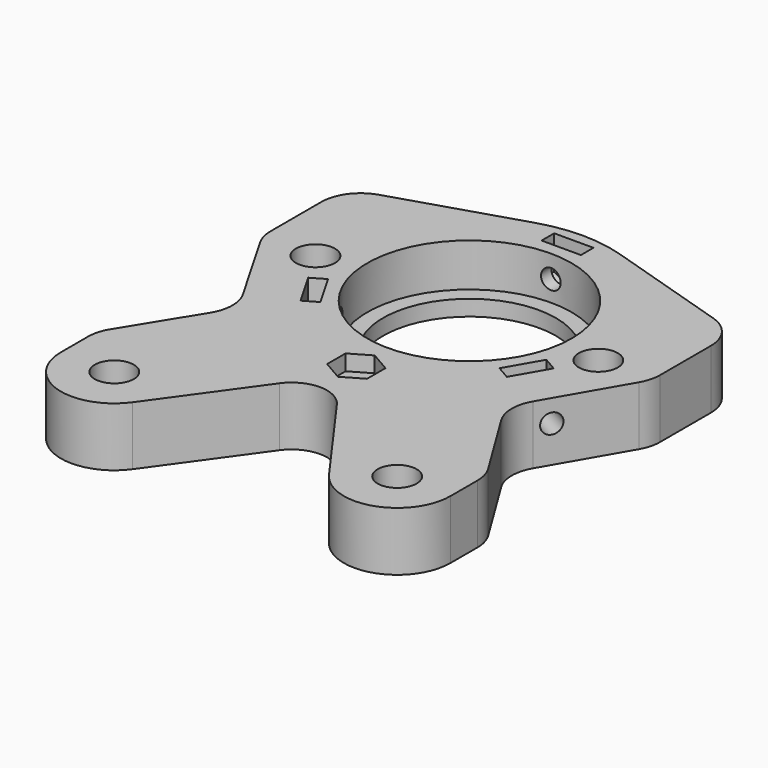
from build123d import *

# Parameters (mm, degrees)
F0_R        = 3.1496
F0_R_2      = 16.51
F1_DEPTH    = 9.525
F0_R_3      = 13.97
F2_DEPTH    = 2.54
F4_DEPTH    = 8.636
F5_T1_DEPTH = 2.54
F5_T3_DEPTH = 2.54
F5_T5_DEPTH = 2.54
F5_T7_DEPTH = 2.54
F5_T9_DEPTH = 2.54
F6_R        = 1.5875
F9_DEPTH    = 5.08
F7_R        = 1.5875
F10_DEPTH   = 20.32
F8_R        = 1.5875
F11_DEPTH   = 20.32
F13_DEPTH   = 2.54


# Not quite as in the source:
# - a fillet or chamfer that OpenCascade refuses, or shapes differently, is made with other operations: its cross-section is extruded or revolved along the edge and cut away or added
# - a feature names something its author has since deleted; it is built from what else it names


with BuildPart() as f1:
    # F0 (on Top) → F1 (new body)
    with BuildSketch(Plane.XY):
        with BuildLine():
            ThreePointArc((6.8331158271, 57.7357942584), (0, 58.780934), (-6.8331158271, 57.7357942584))
            Line((-6.8331158271, 57.7357942584), (-27.0242026981, 51.4112964789))
            ThreePointArc((-27.0242026981, 51.4112964789), (-30.2435047856, 49.1112435687), (-31.4761149683, 45.3516130738))
            Line((-31.4761149683, 45.3516130738), (-31.4761149683, 35.0824113719))
            ThreePointArc((-31.4761149683, 35.0824113719), (-31.2597439653, 33.4389104355), (-30.6253762824, 31.9074113719))
            Line((-30.6253762824, 31.9074113719), (-23.4250291837, 19.436044365))
            ThreePointArc((-23.4250291837, 19.436044365), (-22.5749179632, 16.1717783736), (-23.516459851, 12.9327012793))
            Line((-23.516459851, 12.9327012793), (-30.5339456151, 1.5308194413))
            ThreePointArc((-30.5339456151, 1.5308194413), (-31.2360341416, -0.0679607815), (-31.4761149683, -1.7975236443))
            Line((-31.4761149683, -1.7975236443), (-31.4761149683, -7.259066))
            ThreePointArc((-31.4761149683, -7.259066), (-25.5004563551, -15.4606163037), (-15.8622501042, -12.2858874155))
            Line((-15.8622501042, -12.2858874155), (-4.6415514186, 3.3342503548))
            ThreePointArc((-4.6415514186, 3.3342503548), (0, 5.715), (4.6415514186, 3.3342503548))
            Line((4.6415514186, 3.3342503548), (15.8622501042, -12.2858874155))
            ThreePointArc((15.8622501042, -12.2858874155), (25.5004563551, -15.4606163037), (31.4761149683, -7.259066))
            Line((31.4761149683, -7.259066), (31.4761149683, -1.7975236443))
            ThreePointArc((31.4761149683, -1.7975236443), (31.2360341416, -0.0679607815), (30.5339456151, 1.5308194413))
            Line((30.5339456151, 1.5308194413), (23.516459851, 12.9327012793))
            ThreePointArc((23.516459851, 12.9327012793), (22.5749179632, 16.1717783736), (23.4250291837, 19.436044365))
            Line((23.4250291837, 19.436044365), (30.6253762824, 31.9074113719))
            ThreePointArc((30.6253762824, 31.9074113719), (31.2597439653, 33.4389104355), (31.4761149683, 35.0824113719))
            Line((31.4761149683, 35.0824113719), (31.4761149683, 45.3516130738))
            ThreePointArc((31.4761149683, 45.3516130738), (30.2435047856, 49.1112435687), (27.0242026981, 51.4112964789))
            Line((27.0242026981, 51.4112964789), (6.8331158271, 57.7357942584))
        make_face()
        with Locations((-22.86, -7.259066)):
            Circle(F0_R, mode=Mode.SUBTRACT)
        with Locations((22.86, -7.259066)):
            Circle(F0_R, mode=Mode.SUBTRACT)
        with Locations((-22.86, 33.380934)):
            Circle(F0_R, mode=Mode.SUBTRACT)
        with Locations((0, 35.920934)):
            Circle(F0_R_2, mode=Mode.SUBTRACT)
        with Locations((22.86, 33.380934)):
            Circle(F0_R, mode=Mode.SUBTRACT)
    extrude(amount=F1_DEPTH)

    # F0 (on Top) → F2 (join)
    with BuildSketch(Plane.XY):
        with Locations((0, 35.920934)):
            Circle(F0_R_2)
        with Locations((0, 35.920934)):
            Circle(F0_R_3, mode=Mode.SUBTRACT)
    extrude(amount=F2_DEPTH)

    # F3 (on face) → F4 (cut)
    with BuildSketch(Plane.XY.offset(9.525)):
        Polygon((17.6453415423, 29.39956552), (14.4703415423, 23.900304206), (16.6700460679, 22.630304206), (19.8450460679, 28.12956552), align=None)
        Polygon((-3.175, 57.002932274), (-3.175, 54.462932274), (0, 54.462932274), (3.175, 54.462932274), (3.175, 57.002932274), align=None)
        Polygon((-14.4703415423, 23.900304206), (-17.6453415423, 29.39956552), (-19.8450460679, 28.12956552), (-16.6700460679, 22.630304206), align=None)
    extrude(amount=-F4_DEPTH, mode=Mode.SUBTRACT)

    # F5: chamfer of 3.175 x 5.499261314 on 6 edges, made by hand

    # F5_s2 → F5_t1 (join)
    with BuildSketch(Plane(origin=(-0.5036208564, -0.290765637, 0), x_dir=(0, 0, 1), z_dir=(-0.8660254038, -0.5, 0))):
        Polygon((4.064, 34.2834413717), (0.889, 28.7841800576), (0.889, 34.2834413717), align=None)
    extrude(amount=F5_T1_DEPTH)

    # F5_s4 → F5_t3 (join)
    with BuildSketch(Plane(origin=(-2.703325382, -1.560765637, 0), x_dir=(0, 0, 1), z_dir=(0.8660254038, 0.5, 0))):
        Polygon((4.064, -27.9334413717), (0.889, -33.4327026857), (0.889, -27.9334413717), align=None)
    extrude(amount=F5_T3_DEPTH)

    # F5_s6 → F5_t5 (join)
    with BuildSketch(Plane.XZ.offset(-57.002932274)):
        Polygon((-3.175, 4.064), (2.324261314, 0.889), (-3.175, 0.889), align=None)
        Polygon((3.175, 4.064), (-2.324261314, 0.889), (3.175, 0.889), align=None)
    extrude(amount=F5_T5_DEPTH)

    # F5_s8 → F5_t7 (join)
    with BuildSketch(Plane(origin=(2.703325382, -1.560765637, 0), x_dir=(0, 0, 1), z_dir=(-0.8660254038, 0.5, 0))):
        Polygon((4.064, 34.2834413717), (0.889, 28.7841800576), (0.889, 34.2834413717), align=None)
    extrude(amount=F5_T7_DEPTH)

    # F5_s10 → F5_t9 (join)
    with BuildSketch(Plane(origin=(0.5036208564, -0.290765637, 0), x_dir=(0, 0, 1), z_dir=(0.8660254038, -0.5, 0))):
        Polygon((4.064, -27.9334413717), (0.889, -33.4327026857), (0.889, -27.9334413717), align=None)
    extrude(amount=F5_T9_DEPTH)

    # F6 (on face) → F9 (cut, symmetric)
    with BuildSketch(Plane.XZ.offset(-57.002932274)):
        with Locations((0, 5.8970871047)):
            Circle(F6_R)
    extrude(amount=F9_DEPTH, both=True, mode=Mode.SUBTRACT)

    # F7 (on face) → F10 (cut, symmetric)
    with BuildSketch(Plane(origin=(-2.703325382, -1.560765637, 0), x_dir=(-0.5, 0.8660254038, 0), z_dir=(0.8660254038, 0.5, 0))):
        with Locations((31.0334954411, 5.6098689985)):
            Circle(F7_R)
    extrude(amount=F10_DEPTH, both=True, mode=Mode.SUBTRACT)

    # F8 (on face) → F11 (cut, symmetric)
    with BuildSketch(Plane(origin=(2.703325382, -1.560765637, 0), x_dir=(-0.5, -0.8660254038, 0), z_dir=(-0.8660254038, 0.5, 0))):
        with Locations((-31.1158668548, 5.8928)):
            Circle(F8_R)
    extrude(amount=F11_DEPTH, both=True, mode=Mode.SUBTRACT)

    # F12 (on face) → F13 (cut)
    with BuildSketch(Plane.XY.offset(9.525)):
        Polygon((3.2258, 11.1985175016), (3.2258, 14.9233504984), (0, 16.7857669967), (-3.2258, 14.9233504984), (-3.2258, 11.1985175016), (0, 9.3361010033), align=None)
    extrude(amount=-F13_DEPTH, mode=Mode.SUBTRACT)


with BuildPart() as f14_1:
    # F14: copy of F1
    add(f1.part)


solid = f1.part
